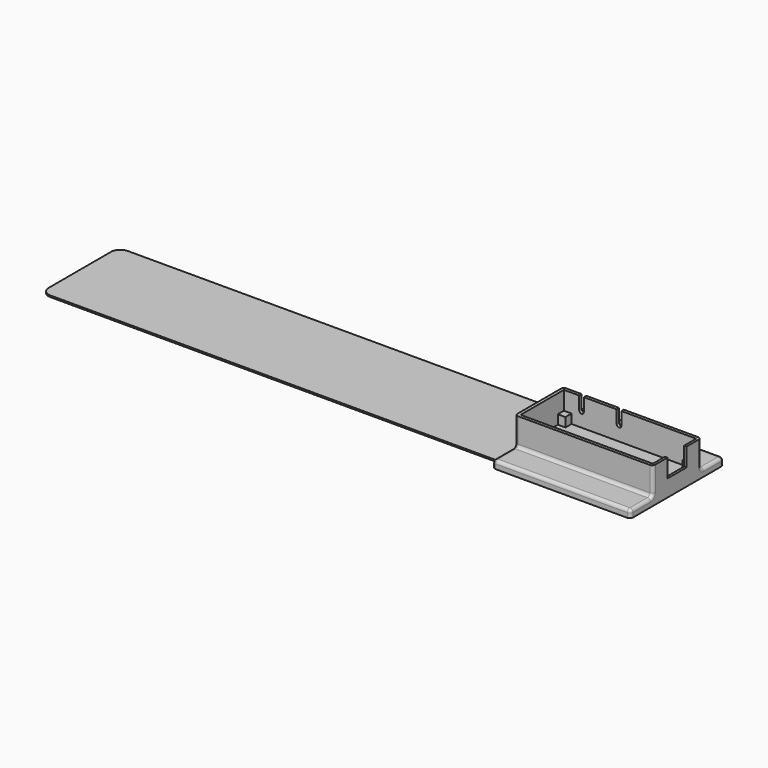
from build123d import *

# Parameters (mm, degrees)
F1_DEPTH  = 0.5
F3_DEPTH  = 2
F4_W      = 45
F4_H      = 19.7
F4_W_2    = 43.2
F4_H_2    = 17.7
F5_DEPTH  = 9
F6_W      = 2.5
F6_H      = 2.5
F7_DEPTH  = 3
F8_W      = 7.8
F8_H      = 6
F9_DEPTH  = 0.8
F10_W     = 1.5
F10_H     = 5
F10_H_2   = 5.0084371828
F11_DEPTH = 1
F12_R     = 0.74999
F13_R     = 1


# Not quite as in the source:
# - a fillet or chamfer is up to 0.001 mm smaller than in the source, because OpenCascade refuses the exact size


with BuildPart() as f1:
    # F0 (on Top) → F1 (new body)
    with BuildSketch(Plane.XY):
        with BuildLine():
            Line((0, -15.75), (0, 15.75))
            Line((0, 15.75), (-147, 15.75))
            ThreePointArc((-147, 15.75), (-149.1213203436, 14.8713203436), (-150, 12.75))
            Line((-150, 12.75), (-150, -12.75))
            ThreePointArc((-150, -12.75), (-149.1213203436, -14.8713203436), (-147, -15.75))
            Line((-147, -15.75), (0, -15.75))
        make_face()
        Polygon((45, 19), (0, 19), (0, 15.75), (0, -15.75), (0, -19), (45, -19), align=None)
    extrude(amount=F1_DEPTH)

    # F2 (on face) → F3 (join)
    with BuildSketch(Plane.XY.offset(0.5)):
        Polygon((45, -19), (45, 19), (0, 19), (0, 15.75), (0, -15.75), (0, -19), align=None)
    extrude(amount=F3_DEPTH)

    # F4 (on face) → F5 (join)
    with BuildSketch(Plane.XY.offset(2.5)):
        with Locations((22.5, 0)):
            Rectangle(F4_W, F4_H)
        with Locations((22.6, 0)):
            Rectangle(F4_W_2, F4_H_2, mode=Mode.SUBTRACT)
    extrude(amount=F5_DEPTH)

    # F6 (on face) → F7 (join)
    with BuildSketch(Plane.XY.offset(2.5)):
        with Locations((2.25, 7.6)):
            Rectangle(F6_W, F6_H)
        with Locations((42.95, 7.6)):
            Rectangle(F6_W, F6_H)
        with Locations((42.95, -7.6)):
            Rectangle(F6_W, F6_H)
        with Locations((2.25, -7.6)):
            Rectangle(F6_W, F6_H)
    extrude(amount=F7_DEPTH)

    # F8 (on face) → F9 (cut, through all)
    with BuildSketch(Plane.YZ.offset(45)):
        with Locations((0, 8.5)):
            Rectangle(F8_W, F8_H)
    extrude(amount=-F9_DEPTH, mode=Mode.SUBTRACT)

    # F10 (on face) → F11 (cut, through all)
    with BuildSketch(Plane(origin=(0, 9.85, 0), x_dir=(-1, 0, 0), z_dir=(0, 1, 0))):
        with Locations((-19, 9)):
            Rectangle(F10_W, F10_H)
        with Locations((-6.75, 8.9957814086)):
            Rectangle(F10_W, F10_H_2)
    extrude(amount=-F11_DEPTH, mode=Mode.SUBTRACT)

    # F12 (radius 0.75 in the source; OpenCascade refuses exactly that, so slightly less here)
    f12_edges = [f1.edges().sort_by_distance(p)[0] for p in [
        (18.25, 9.35, 6.5),
        (19.75, 9.35, 6.5),
        (6, 9.35, 6.491563),
        (7.5, 9.35, 6.491563),
    ]]
    fillet(f12_edges, radius=F12_R)

    # F13
    f13_edges = [f1.edges().sort_by_distance(p)[0] for p in [
        (45, 9.85, 7),
        (45, 14.425, 2.5),
        (45, 19, 1.25),
        (22.5, 19, 2.5),
        (0, 14.425, 2.5),
        (0, 9.85, 7),
        (22.5, 9.85, 2.5),
        (0, -9.85, 7),
        (0, -14.425, 2.5),
        (0, -19, 1.25),
        (22.5, -19, 2.5),
        (22.5, -9.85, 2.5),
        (45, -9.85, 7),
        (45, -14.425, 2.5),
        (45, -19, 1.25),
        (0, 19, 1.25),
    ]]
    fillet(f13_edges, radius=F13_R)


solid = f1.part
